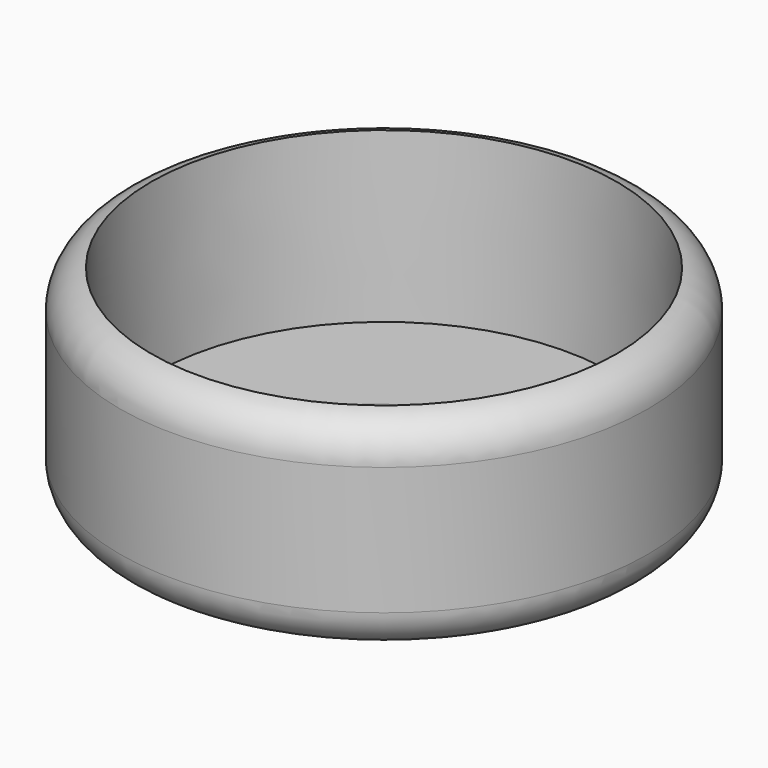
from build123d import *


# Not quite as in the source:
# - a fillet or chamfer that OpenCascade refuses, or shapes differently, is made with other operations: its cross-section is extruded or revolved along the edge and cut away or added


with BuildPart() as f1:
    # F0 (on Front) → F1 (revolve)
    with BuildSketch(Plane.XZ):
        Polygon((-13.5, 0), (0, 0), (0, 2), (-11.65, 2), (-13.5, 2), align=None)
        Polygon((-13.5, 10.5), (-13.5, 2), (-11.65, 2), (-11.9, 10.5), align=None)
    revolve(axis=Axis((0, 0, 1), (0, 0, 1)))

    # F2: fillet of radius 2 on 2 edges, made by hand

    # F2_s1 → F2_t2 (revolve, cut)
    with BuildSketch(Plane.XZ):
        with BuildLine():
            ThreePointArc((-11.9, 10.5), (-13.0491933385, 9.8053192698), (-13.5, 8.5404082058))
            Line((-13.5, 8.5404082058), (-13.5, 10.5))
            Line((-13.5, 10.5), (-11.9, 10.5))
        make_face()
    revolve(axis=Axis((0, 0, 10.5), (0, 0, 1)), mode=Mode.SUBTRACT)

    # F2_s3 → F2_t4 (revolve, cut)
    with BuildSketch(Plane.XZ):
        with BuildLine():
            ThreePointArc((-11.5, 0), (-12.9142135624, 0.5857864376), (-13.5, 2))
            Line((-13.5, 2), (-13.5, 0))
            Line((-13.5, 0), (-11.5, 0))
        make_face()
    revolve(axis=Axis((0, 0, 0), (0, 0, 1)), mode=Mode.SUBTRACT)

    # F3 (on Front) → F4 (revolve, cut)
    with BuildSketch(Plane.XZ):
        with BuildLine():
            Line((11.7787091929, 11.2052995105), (-11.8056663253, 11.404592826))
            ThreePointArc((-11.8056663253, 11.404592826), (-0.1005541056, 1.0004248449), (11.7787091929, 11.2052995105))
        make_face()
    revolve(axis=Axis((-0.0134785662, 0, 11.3049461682), (0.9999642987, 0, -0.0084499248)), mode=Mode.SUBTRACT)


solid = f1.part
